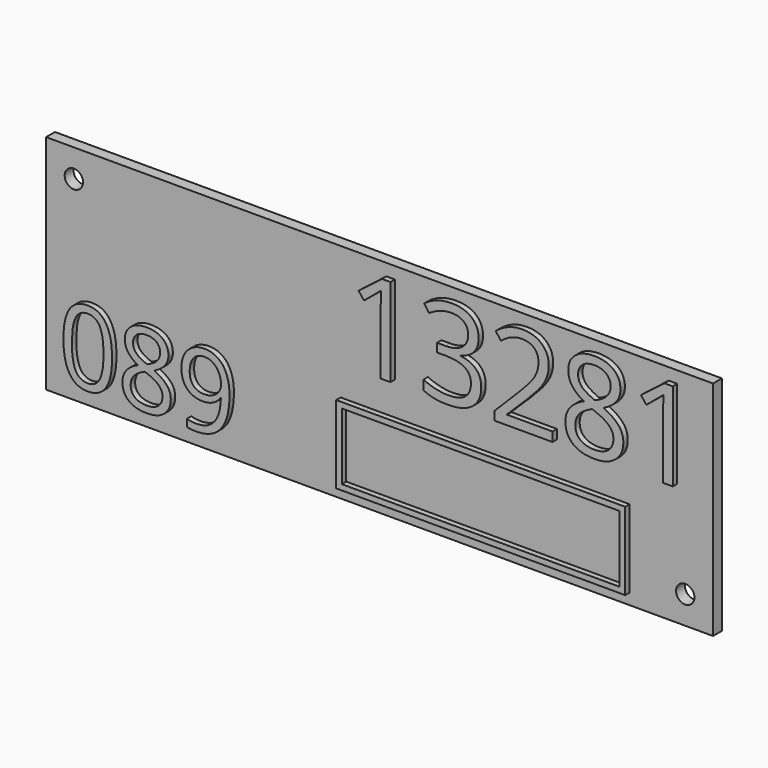
from build123d import *

# Parameters (mm, degrees)
F0_W         = 120
F0_H         = 40
F1_DEPTH     = 2
F3_D         = 3.3
F4_TEXT_SIZE = 22.2157940411
F5_DEPTH     = 1
F6_TEXT_SIZE = 18.5356140827
F7_DEPTH     = 1
F8_W         = 52
F8_H         = 14
F8_W_2       = 49.99999962
F8_H_2       = 11.99999962
F9_DEPTH     = 1


# Not quite as in the source:
# - Text() gives the source's letters only with a copy of the font that has no kerning and outlines rounded to 1/6400 em; it was checked with that copy


with BuildPart() as f1:
    # F0 (on Front) → F1 (new body)
    with BuildSketch(Plane.XZ):
        Rectangle(F0_W, F0_H)
    extrude(amount=F1_DEPTH)

    # F3 (through all)
    with Locations(Plane.XZ.offset(2)):
        with Locations((-55, 15), (55, -15)):
            Hole(F3_D / 2)

    # F4 (on face) → F5 (join)
    with BuildSketch(Plane.XZ.offset(2)):
        with Locations((-5, 2)):
            Text('13281', F4_TEXT_SIZE, font='Open Sans', text_align=(TextAlign.LEFT, TextAlign.BOTTOM))
    extrude(amount=F5_DEPTH)

    # F6 (on face) → F7 (join)
    with BuildSketch(Plane.XZ.offset(2)):
        with Locations((-57, -17)):
            Text('089', F6_TEXT_SIZE, font='Open Sans', text_align=(TextAlign.LEFT, TextAlign.BOTTOM))
    extrude(amount=F7_DEPTH)

    # F8 (on face) → F9 (join)
    with BuildSketch(Plane.XZ.offset(2)):
        with Locations((19, -11)):
            Rectangle(F8_W, F8_H)
        with Locations((19, -11)):
            Rectangle(F8_W_2, F8_H_2, mode=Mode.SUBTRACT)
    extrude(amount=F9_DEPTH)


solid = f1.part
